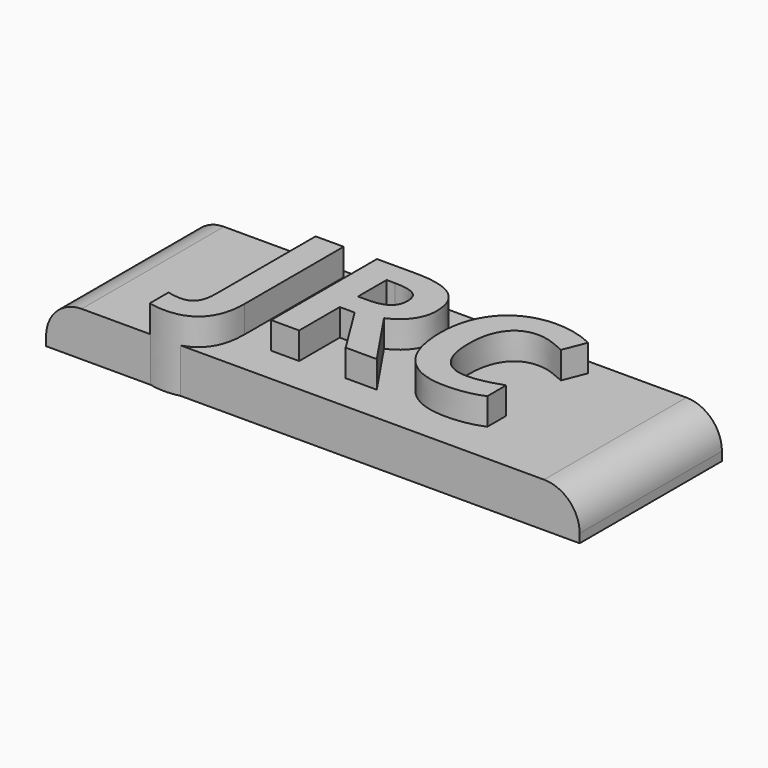
from build123d import *

# Parameters (mm, degrees)
F0_W         = 76.2
F0_H         = 25.4
F1_DEPTH     = 6.35
F2_TEXT_SIZE = 26.4583333333
F3_DEPTH     = 10.198
F4_R         = 5.08


# Not quite as in the source:
# - Text() gives the source's letters only with a copy of the font that has no kerning and outlines rounded to 1/6400 em; it was checked with that copy


with BuildPart() as f1:
    # F0 (on Top) → F1 (new body)
    with BuildSketch(Plane.XY):
        Rectangle(F0_W, F0_H)
    extrude(amount=F1_DEPTH)

    # F2 (on Top) → F3 (join)
    with BuildSketch(Plane.XY):
        with Locations((-21.34518437, -7.3923543755)):
            Text('JRC', F2_TEXT_SIZE, font='Open Sans', font_style=FontStyle.BOLD, text_align=(TextAlign.LEFT, TextAlign.BOTTOM))
    extrude(amount=F3_DEPTH)

    # F4
    f4_edges = [f1.edges().sort_by_distance(p)[0] for p in [
        (-38.1, 0, 6.35),
        (38.1, 0, 6.35),
    ]]
    fillet(f4_edges, radius=F4_R)


solid = f1.part
